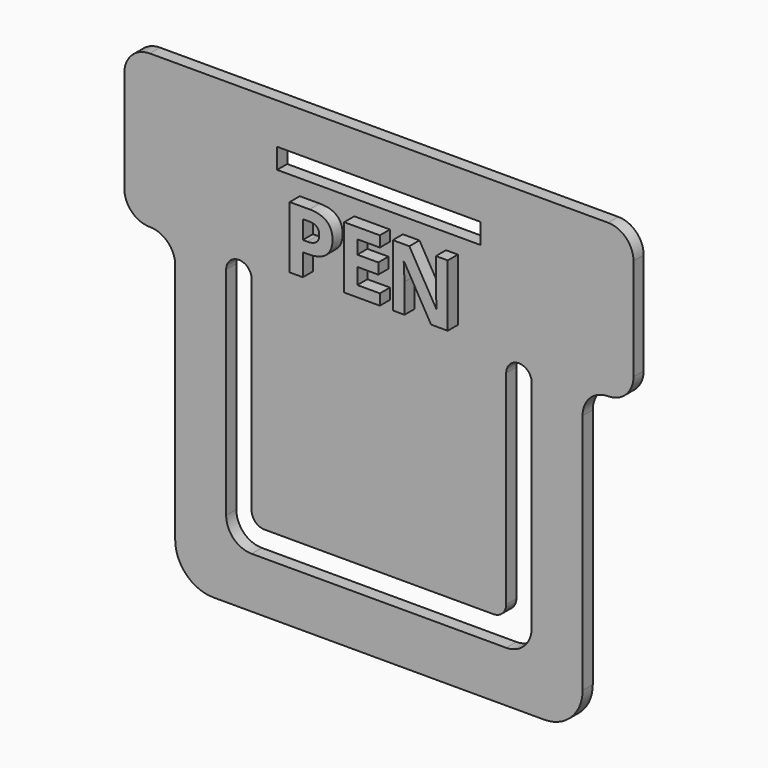
from build123d import *

# Parameters (mm, degrees)
F0_W          = 25.4
F0_H          = 19.05
F1_DEPTH      = 0.79375
F2_R          = 2.38125
F3_W          = 19.05
F3_H          = 15.875
F4_DEPTH      = 4.9276
F5_W          = 12.7
F5_H          = 1.27
F6_DEPTH      = 0.79375
F7_R          = 1.58749
F8_R          = 1.5875
F9_W          = 12.7
F9_H          = 1.27
F9_W_2        = 15.875
F9_H_2        = 14.2875
F10_DEPTH     = 0.79375
F11_R         = 0.79374
F12_R         = 0.79375
F13_TEXT_SIZE = 5.4105680519
F14_DEPTH     = 0.7874


# Not quite as in the source:
# - a fillet or chamfer is up to 0.001 mm smaller than in the source, because OpenCascade refuses the exact size
# - ends of sketch curves that miss each other by under 0.0002 mm in the source are joined
# - Text() gives the source's letters only with a copy of the font that has no kerning and outlines rounded to 1/6400 em; it was checked with that copy


with BuildPart() as f1:
    # F0 (on Front) → F1 (new body)
    with BuildSketch(Plane.XZ):
        Rectangle(F0_W, F0_H)
    extrude(amount=F1_DEPTH)

    # F2
    f2_edges = [f1.edges().sort_by_distance(p)[0] for p in [
        (12.7, -0.396875, -9.525),
        (-12.7, -0.396875, -9.525),
    ]]
    fillet(f2_edges, radius=F2_R)

    # F3 (on face) → F4 (cut)
    with BuildSketch(Plane.XZ.offset(0.79375)):
        with Locations((0, 1.5875)):
            Rectangle(F3_W, F3_H)
    extrude(amount=-F4_DEPTH, mode=Mode.SUBTRACT)

    # F5 (on face) → F6 (join)
    with BuildSketch(Plane.XZ.offset(0.79375)):
        Polygon((-15.875, 19.05), (-15.875, 9.525), (-12.7, 9.525), (-9.525, 9.525), (9.525, 9.525), (12.7, 9.525), (15.875, 9.525), (15.875, 19.05), align=None)
        with Locations((0, 15.875)):
            Rectangle(F5_W, F5_H, mode=Mode.SUBTRACT)
    extrude(amount=-F6_DEPTH)

    # F7 (radius 1.5875 in the source; OpenCascade refuses exactly that, so slightly less here)
    f7_edges = [f1.edges().sort_by_distance(p)[0] for p in [
        (-15.875, -0.396875, 19.05),
        (15.875, -0.396875, 19.05),
        (15.875, -0.396875, 9.525),
        (12.7, -0.396875, 9.525),
        (-15.875, -0.396875, 9.525),
        (-12.7, -0.396875, 9.525),
    ]]
    fillet(f7_edges, radius=F7_R)

    # F8
    f8_edges = [f1.edges().sort_by_distance(p)[0] for p in [
        (-9.525, -0.396875, -6.35),
        (9.525, -0.396875, -6.35),
    ]]
    fillet(f8_edges, radius=F8_R)

    # F9 (on face) → F10 (join)
    with BuildSketch(Plane.XZ.offset(0.79375)):
        with BuildLine():
            ThreePointArc((-14.28751, 19.05), (-15.4100349441, 18.5850349441), (-15.875, 17.46251))
            Line((-15.875, 17.46251), (-15.875, 11.11249))
            ThreePointArc((-15.875, 11.11249), (-15.4100349441, 9.9899650559), (-14.28751, 9.525))
            ThreePointArc((-14.28751, 9.525), (-13.1649650559, 9.0600349441), (-12.7, 7.93751))
            Line((-12.7, 7.93751), (-12.7, -7.14375))
            ThreePointArc((-12.7, -7.14375), (-12.0025480227, -8.8275480227), (-10.31875, -9.525))
            Line((-10.31875, -9.525), (10.31875, -9.525))
            ThreePointArc((10.31875, -9.525), (12.0025480227, -8.8275480227), (12.7, -7.14375))
            Line((12.7, -7.14375), (12.7, 7.93751))
            ThreePointArc((12.7, 7.93751), (13.1649650559, 9.0600349441), (14.28749, 9.525))
            ThreePointArc((14.28749, 9.525), (15.4100349441, 9.9899650559), (15.875, 11.11249))
            Line((15.875, 11.11249), (15.875, 17.46251))
            ThreePointArc((15.875, 17.46251), (15.4100349441, 18.5850349441), (14.28751, 19.05))
            Line((14.28751, 19.05), (-14.28751, 19.05))
        make_face()
        with BuildLine():
            Line((-9.525, 9.525), (-7.9375, 9.525))
            Line((-7.9375, 9.525), (7.9375, 9.525))
            Line((7.9375, 9.525), (9.525, 9.525))
            Line((9.525, 9.525), (9.525, -4.7625))
            ThreePointArc((9.525, -4.7625), (9.0600320151, -5.8850320151), (7.9375, -6.35))
            Line((7.9375, -6.35), (-7.9375, -6.35))
            ThreePointArc((-7.9375, -6.35), (-9.0600320151, -5.8850320151), (-9.525, -4.7625))
            Line((-9.525, -4.7625), (-9.525, 9.525))
        make_face(mode=Mode.SUBTRACT)
        with Locations((0, 15.875)):
            Rectangle(F9_W, F9_H, mode=Mode.SUBTRACT)
        with Locations((0, 2.38125)):
            Rectangle(F9_W_2, F9_H_2)
    extrude(amount=-F10_DEPTH)

    # F11 (radius 0.79375 in the source; OpenCascade refuses exactly that, so slightly less here)
    f11_edges = [f1.edges().sort_by_distance(p)[0] for p in [
        (-7.9375, -0.396875, 9.525),
        (-9.525, -0.396875, 9.525),
        (7.9375, -0.396875, 9.525),
        (9.525, -0.396875, 9.525),
    ]]
    fillet(f11_edges, radius=F11_R)

    # F12
    f12_edges = [f1.edges().sort_by_distance(p)[0] for p in [
        (-7.9375, -0.396875, -4.7625),
        (7.9375, -0.396875, -4.7625),
    ]]
    fillet(f12_edges, radius=F12_R)

    # F13 (on face) → F14 (join)
    with BuildSketch(Plane.XZ.offset(0.79375)):
        with Locations((-5.4185616318, 10.3918910027)):
            Text('PEN', F13_TEXT_SIZE, font='Open Sans', font_style=FontStyle.BOLD, text_align=(TextAlign.LEFT, TextAlign.BOTTOM))
    extrude(amount=F14_DEPTH)


solid = f1.part
